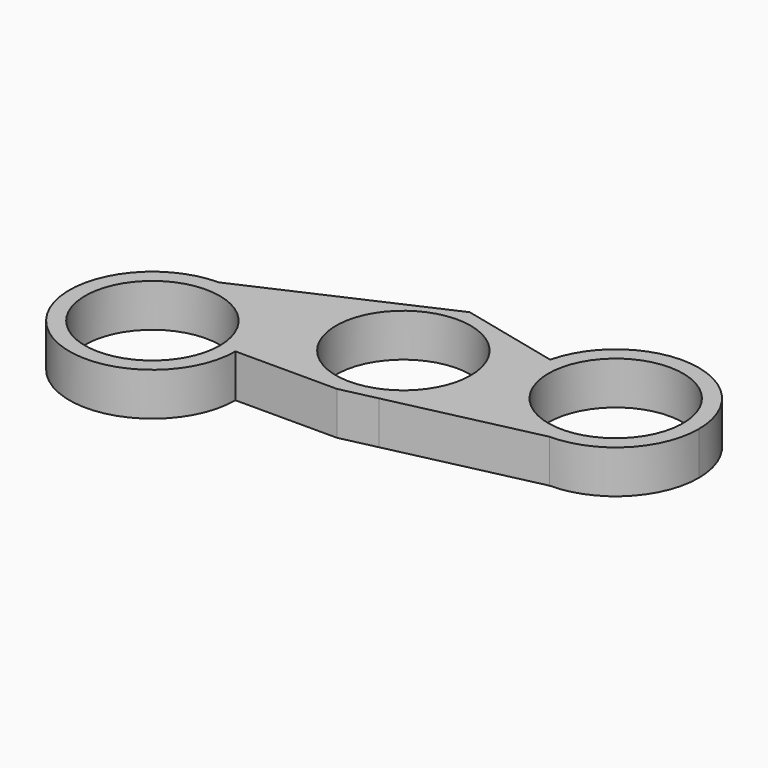
from build123d import *

# Parameters (mm, degrees)
F0_R     = 10.95
F1_DEPTH = 7


# Not quite as in the source:
# - a feature names something its author has since deleted; it is built from what else it names


with BuildPart() as f1:
    # F0 (on Top) → F1 (new body)
    with BuildSketch(Plane.XY):
        with BuildLine():
            ThreePointArc((-56.191941013, 7.2029190708), (-65.7378825591, -15.8430224752), (-42.691941013, -6.2970809292))
            ThreePointArc((-42.691941013, -6.2970809292), (-46.645999467, 3.2488606168), (-56.191941013, 7.2029190708))
        make_face()
        with Locations((-56.191941013, -6.2970809292)):
            Circle(F0_R, mode=Mode.SUBTRACT)
        with BuildLine():
            Line((-42.691941013, -6.2970809292), (-26.191941013, -6.2970809292))
            ThreePointArc((-26.191941013, -6.2970809292), (-38.5028813329, 1.6629959269), (-36.295891117, 16.156141524))
            Line((-36.295891117, 16.156141524), (-56.191941013, 7.2029190708))
            ThreePointArc((-56.191941013, 7.2029190708), (-46.645999467, 3.2488606168), (-42.691941013, -6.2970809292))
        make_face()
        with BuildLine():
            ThreePointArc((-20.4170961141, -4.9995874911), (-14.7855742353, -0.0182163615), (-12.691941013, 7.2029190708))
            ThreePointArc((-12.691941013, 7.2029190708), (-14.704995322, 14.295173909), (-20.1438045227, 19.2723036862))
            Line((-20.1438045227, 19.2723036862), (-26.191941013, 20.7029190708))
            Line((-26.191941013, 20.7029190708), (-36.295891117, 16.156141524))
            ThreePointArc((-36.295891117, 16.156141524), (-38.5028813329, 1.6629959269), (-26.191941013, -6.2970809292))
            Line((-26.191941013, -6.2970809292), (-20.4170961141, -4.9995874911))
        make_face()
        with Locations((-26.191941013, 7.2029190708)):
            Circle(F0_R, mode=Mode.SUBTRACT)
        with BuildLine():
            ThreePointArc((-20.1438045227, 19.2723036862), (-14.704995322, 14.295173909), (-12.691941013, 7.2029190708))
            ThreePointArc((-12.691941013, 7.2029190708), (-14.7855742353, -0.0182163615), (-20.4170961141, -4.9995874911))
            Line((-20.4170961141, -4.9995874911), (3.0783548298, 0.27937566))
            ThreePointArc((3.0783548298, 0.27937566), (-7.5094084371, 5.4038596161), (-10.0591238534, 16.8868913633))
            Line((-10.0591238534, 16.8868913633), (-20.1438045227, 19.2723036862))
        make_face()
        with BuildLine():
            ThreePointArc((16.5783548298, 13.77937566), (4.6426498429, 27.1884390543), (-10.0591238534, 16.8868913633))
            ThreePointArc((-10.0591238534, 16.8868913633), (-7.5094084371, 5.4038596161), (3.0783548298, 0.27937566))
            ThreePointArc((3.0783548298, 0.27937566), (12.6242963759, 4.233434114), (16.5783548298, 13.77937566))
        make_face()
        with BuildLine():
            ThreePointArc((14.0283548298, 13.77937566), (1.8095377637, 2.9031353513), (-7.5776001022, 16.2999161749))
            ThreePointArc((-7.5776001022, 16.2999161749), (4.347171896, 24.6556159687), (14.0283548298, 13.77937566))
        make_face(mode=Mode.SUBTRACT)
    extrude(amount=F1_DEPTH)


solid = f1.part
